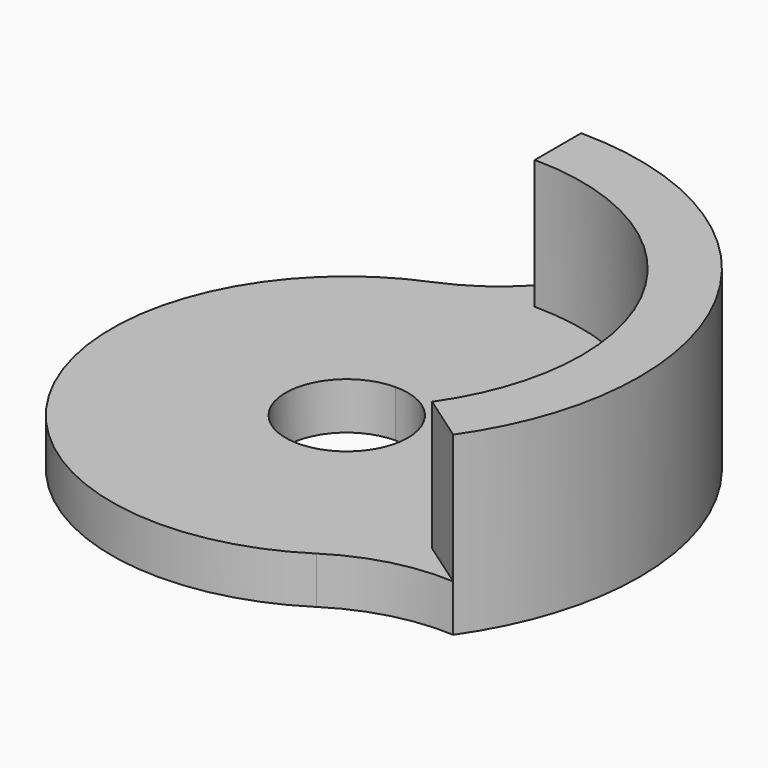
from build123d import *

# Parameters (mm, degrees)
F1_DEPTH    = 1.27
F2_DEPTH    = 4.7625
F3_T1_DEPTH = 1.27


# Not quite as in the source:
# - a fillet or chamfer that OpenCascade refuses, or shapes differently, is made with other operations: its cross-section is extruded or revolved along the edge and cut away or added
# - a feature names something its author has since deleted; it is built from what else it names


with BuildPart() as f1:
    # F0 (on Top) → F1 (new body)
    with BuildSketch(Plane.XY):
        with BuildLine():
            ThreePointArc((5.2108397025, -3.6290011842), (6.0585201209, -1.9017975562), (6.35, 0))
            ThreePointArc((6.35, 0), (4.4901280605, 4.4901280605), (0, 6.35))
            Line((0, 6.35), (0, 5.1572436072))
            ThreePointArc((0, 5.1572436072), (3.6467219269, 3.6467219269), (5.1572436072, 0))
            ThreePointArc((5.1572436072, 0), (4.9205140413, -1.5445721714), (4.2320582273, -2.9473453792))
            Line((4.2320582273, -2.9473453792), (5.2108397025, -3.6290011842))
        make_face()
        with BuildLine():
            ThreePointArc((0, 6.35), (4.4901280605, 4.4901280605), (6.35, 0))
            ThreePointArc((6.35, 0), (6.0585201209, -1.9017975562), (5.2108397025, -3.6290011842))
            Line((5.2108397025, -3.6290011842), (6.4969090936, -4.5246624615))
            ThreePointArc((6.4969090936, -4.5246624615), (7.5538025952, -2.3711736577), (7.9172216188, 0))
            ThreePointArc((7.9172216188, 0), (5.5983210948, 5.5983210948), (0, 7.9172216188))
            Line((0, 7.9172216188), (0, 6.35))
        make_face()
        with BuildLine():
            Line((0, 5.1572436072), (0, 6.35))
            ThreePointArc((0, 6.35), (-5.6287946099, -2.939246713), (5.2108397025, -3.6290011842))
            Line((5.2108397025, -3.6290011842), (4.2320582273, -2.9473453792))
            ThreePointArc((4.2320582273, -2.9473453792), (-4.571506302, -2.3871513891), (0, 5.1572436072))
        make_face()
        with BuildLine():
            Line((0, 1.651), (0, 5.1572436072))
            ThreePointArc((0, 5.1572436072), (-4.571506302, -2.3871513891), (4.2320582273, -2.9473453792))
            Line((4.2320582273, -2.9473453792), (1.3548183226, -0.9435403079))
            ThreePointArc((1.3548183226, -0.9435403079), (-1.4634865986, -0.7642041454), (0, 1.651))
        make_face()
        with BuildLine():
            ThreePointArc((5.1572436072, 0), (3.6467219269, 3.6467219269), (0, 5.1572436072))
            Line((0, 5.1572436072), (0, 1.651))
            ThreePointArc((0, 1.651), (1.1674332957, 1.1674332957), (1.651, 0))
            ThreePointArc((1.651, 0), (1.5752152314, -0.4944673646), (1.3548183226, -0.9435403079))
            Line((1.3548183226, -0.9435403079), (4.2320582273, -2.9473453792))
            ThreePointArc((4.2320582273, -2.9473453792), (4.9205140413, -1.5445721714), (5.1572436072, 0))
        make_face()
    extrude(amount=F1_DEPTH)

    # F0 (on Top) → F2 (join)
    with BuildSketch(Plane.XY):
        with BuildLine():
            ThreePointArc((0, 6.35), (4.4901280605, 4.4901280605), (6.35, 0))
            ThreePointArc((6.35, 0), (6.0585201209, -1.9017975562), (5.2108397025, -3.6290011842))
            Line((5.2108397025, -3.6290011842), (6.4969090936, -4.5246624615))
            ThreePointArc((6.4969090936, -4.5246624615), (7.5538025952, -2.3711736577), (7.9172216188, 0))
            ThreePointArc((7.9172216188, 0), (5.5983210948, 5.5983210948), (0, 7.9172216188))
            Line((0, 7.9172216188), (0, 6.35))
        make_face()
    extrude(amount=F2_DEPTH)

    # F3: fillet of radius 5.08 on 2 edges, made by hand

    # F3_s2 → F3_t1 (join)
    with BuildSketch(Plane.XY):
        with BuildLine():
            ThreePointArc((0, 7.9172216188), (-1.0395816291, 6.7062044575), (-2.4036069424, 5.8775142421))
            ThreePointArc((-2.4036069424, 5.8775142421), (-1.2248029561, 6.2307590002), (0, 6.35))
            Line((0, 6.35), (0, 7.9172216188))
        make_face()
        with BuildLine():
            ThreePointArc((6.4969090936, -4.5246624615), (4.9090257444, -4.6856562433), (3.4494633266, -5.3313884456))
            ThreePointArc((3.4494633266, -5.3313884456), (4.4130196845, -4.5659344349), (5.2108397025, -3.6290011842))
            Line((5.2108397025, -3.6290011842), (6.4969090936, -4.5246624615))
        make_face()
    extrude(amount=F3_T1_DEPTH)


solid = f1.part
